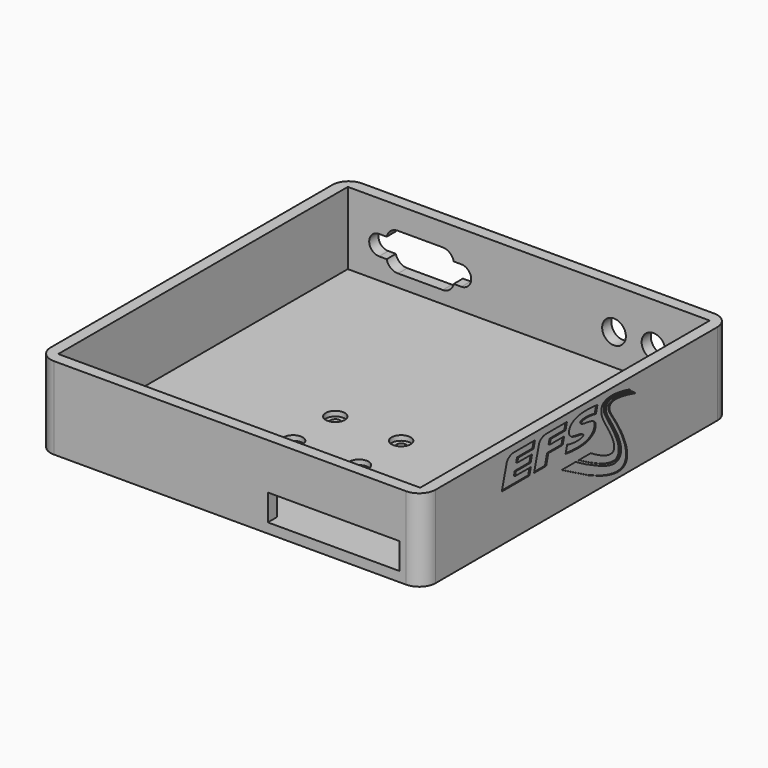
from build123d import *

# Parameters (mm, degrees)
F0_W      = 117
F0_H      = 117
F0_W_2    = 110
F0_H_2    = 110
F1_DEPTH  = 25
F2_DEPTH  = 3
F3_R      = 5
F4_R      = 5
F5_R      = 5
F7_R      = 3.6
F8_DEPTH  = 8.5856
F9_W      = 40
F9_H      = 8
F10_DEPTH = 25
F11_R     = 1.5
F12_DEPTH = 3
F13_R     = 2.9
F14_DEPTH = 1.5
F17_DEPTH = 2
F18_SCALE = 0.2


# Not quite as in the source:
# - two fillets or chamfers of one size are made in one step
# - a feature names something its author has since deleted; it is built from what else it names


with BuildPart() as f1:
    # F0 (on Top) → F1 (new body)
    with BuildSketch(Plane.XY):
        with Locations((0, 23.8324391609)):
            Rectangle(F0_W, F0_H)
        with Locations((0, 23.8324391609)):
            Rectangle(F0_W_2, F0_H_2, mode=Mode.SUBTRACT)
    extrude(amount=F1_DEPTH)

    # F0 (on Top) → F2 (join)
    with BuildSketch(Plane.XY):
        with Locations((0, 23.8324391609)):
            Rectangle(F0_W_2, F0_H_2)
    extrude(amount=F2_DEPTH)

    # F3
    f3_edges = [f1.edges().sort_by_distance(p)[0] for p in [
        (58.5, -34.667561, 12.5),
    ]]
    fillet(f3_edges, radius=F3_R)

    # F4
    f4_edges = [f1.edges().sort_by_distance(p)[0] for p in [
        (-58.5, -34.667561, 12.5),
    ]]
    fillet(f4_edges, radius=F4_R)

    # F5
    f5_edges = [f1.edges().sort_by_distance(p)[0] for p in [
        (58.5, 82.332439, 12.5),
        (-58.5, 82.332439, 12.5),
    ]]
    fillet(f5_edges, radius=F5_R)

    # F7 (on face) → F8 (cut)
    with BuildSketch(Plane(origin=(0, 82.3324391609, 0), x_dir=(-1, 0, 0), z_dir=(0, 1, 0))):
        with BuildLine():
            Line((39.85, 18.2), (26.15, 18.2))
            ThreePointArc((26.15, 18.2), (24.0075714714, 17.4400757565), (22.8228390481, 15.5))
            Line((22.8228390481, 15.5), (20.5, 15.5))
            ThreePointArc((20.5, 15.5), (17.5, 12.5), (20.5, 9.5))
            Line((20.5, 9.5), (22.8228390481, 9.5))
            ThreePointArc((22.8228390481, 9.5), (24.0075714714, 7.5599242435), (26.15, 6.8))
            Line((26.15, 6.8), (39.7201597989, 6.8))
            ThreePointArc((39.7201597989, 6.8), (41.9426174229, 7.5177900105), (43.1776817724, 9.5))
            Line((43.1776817724, 9.5), (45.5, 9.5))
            ThreePointArc((45.5, 9.5), (48.5, 12.5), (45.5, 15.5))
            ThreePointArc((45.5, 15.5), (44.2542750291, 15.2291334333), (43.2335002222, 14.465446198))
            ThreePointArc((43.2335002222, 14.465446198), (43.2449696229, 14.984881744), (43.1771609519, 15.5))
            ThreePointArc((43.1771609519, 15.5), (41.9924285286, 17.4400757565), (39.85, 18.2))
        make_face()
        with BuildLine():
            Line((45.5, 15.5), (43.1771609519, 15.5))
            ThreePointArc((43.1771609519, 15.5), (43.2449696229, 14.984881744), (43.2335002222, 14.465446198))
            ThreePointArc((43.2335002222, 14.465446198), (44.2542750291, 15.2291334333), (45.5, 15.5))
        make_face()
        with Locations((-37.9, 12.5)):
            Circle(F7_R)
        with Locations((-25.9, 12.5)):
            Circle(F7_R)
    extrude(amount=-F8_DEPTH, mode=Mode.SUBTRACT)

    # F9 (on face) → F10 (cut)
    with BuildSketch(Plane.XZ.offset(34.6675608391)):
        with Locations((31.5, 7)):
            Rectangle(F9_W, F9_H)
    extrude(amount=-F10_DEPTH, mode=Mode.SUBTRACT)

    # F11 (on face) → F12 (cut, through all)
    with BuildSketch(Plane(origin=(0, 0, 0), x_dir=(1, 0, 0), z_dir=(0, 0, -1))):
        with Locations((-10, -1.8324391609)):
            Circle(F11_R)
        with Locations((10, -1.8324391609)):
            Circle(F11_R)
        with Locations((10, -17.8324391609)):
            Circle(F11_R)
        with Locations((-10, -17.8324391609)):
            Circle(F11_R)
    extrude(amount=-F12_DEPTH, mode=Mode.SUBTRACT)

    # F13 (on face) → F14 (cut)
    with BuildSketch(Plane.XY.offset(3)):
        with Locations((-10, 17.8324391609)):
            Circle(F13_R)
        with Locations((10, 17.8324391609)):
            Circle(F13_R)
        with Locations((10, 1.8324391609)):
            Circle(F13_R)
        with Locations((-10, 1.8324391609)):
            Circle(F13_R)
    extrude(amount=-F14_DEPTH, mode=Mode.SUBTRACT)


with BuildPart() as f17:
    # F16 (on face) → F17 (new body)
    with BuildSketch(Plane.YZ.offset(58.5)):
        Polygon((-66.8057338, 42.572559), (-64.087883, 52.9304758), (-103.1221458, 52.9304758), (-105.1262312, 52.8319492), (-106.9472588, 52.599463), (-108.5937376, 52.2488668), (-110.0742782, 51.7959594), (-111.397415, 51.2566158), (-112.0026462, 50.9594866), (-112.5717078, 50.6466856), (-113.1057174, 50.3201686), (-113.605691, 49.9819676), (-114.5079498, 49.2783368), (-115.2869932, 48.5516174), (-115.9514064, 47.817659), (-116.5097492, 47.0922858), (-116.9705306, 46.3913728), (-117.3423612, 45.7307188), (-117.6337754, 45.1261988), (-117.8533076, 44.5936116), (-118.0095176, 44.1488576), (-127, 9.8964496), (-74.7851946, 9.8964496), (-72.0665818, 20.254341), (-101.9276346, 20.254341), (-100.3902996, 26.1122922), (-72.406383, 26.1122922), (-69.6877702, 36.469447), (-97.6724742, 36.469447), (-96.0704454, 42.572559), align=None)
    extrude(amount=F17_DEPTH)


with BuildPart() as f17b:
    # F16 (on face) → F17, piece 2 (new body)
    with BuildSketch(Plane.YZ.offset(58.5)):
        Polygon((-43.0960671327, 52.859241217), (-44.9142245327, 52.685556017), (-46.5680947327, 52.396834217), (-48.0652977327, 52.007071217), (-49.4133773327, 51.530287817), (-50.6199281327, 50.980530217), (-51.6925193327, 50.371819217), (-52.6387455327, 49.718175617), (-53.4661759327, 49.033620217), (-54.1824051327, 48.332199217), (-54.7950023327, 47.627908017), (-55.3115113327, 46.934818217), (-55.7395775327, 46.266925217), (-56.0867193327, 45.638275217), (-56.3605567327, 45.062863617), (-56.5686335327, 44.554736617), (-56.7185697327, 44.127940417), (-65.7222855327, 9.825215017), (-42.8577135327, 9.825215017), (-38.8280543327, 25.176848017), (-11.5263309327, 25.176848017), (-8.8073371327, 35.534764817), (-36.1094669327, 35.534764817), (-34.2811749327, 42.501324417), (-6.1265957327, 42.501324417), (-3.4072463327, 52.859241217), align=None)
    extrude(amount=F17_DEPTH)


with BuildPart() as f17c:
    # F16 (on face) → F17, piece 3 (new body)
    with BuildSketch(Plane.YZ.offset(58.5)):
        Polygon((24.8065699738, 38.5670330833), (24.6279825738, 38.6749830833), (24.4689531738, 38.7889782833), (24.3967917738, 38.8482110833), (24.3295071738, 38.9089678833), (24.2670993738, 38.9712486833), (24.2096191738, 39.0350026833), (24.1569903738, 39.1002806833), (24.1092891738, 39.1670826833), (24.0664647738, 39.2353832833), (24.0285425738, 39.3051824833), (23.9955225738, 39.3764802833), (23.9673793738, 39.4493020833), (23.9441383738, 39.5236224833), (23.9257995738, 39.5994668833), (23.9123629738, 39.6768098833), (23.9038285738, 39.7556768833), (23.9001709738, 39.8360424833), (23.9014155738, 39.9179320833), (23.9075877738, 40.0013202833), (23.9186367738, 40.0862070833), (23.9345879738, 40.1726432833), (23.9554413738, 40.2605526833), (23.9932111738, 40.3896608833), (24.0379913738, 40.5149336833), (24.0897565738, 40.6363456833), (24.1485321738, 40.7538968833), (24.2143181738, 40.8676126833), (24.2870891738, 40.9774930833), (24.3668705738, 41.0835126833), (24.4536623738, 41.1856714833), (24.5474391738, 41.2839948833), (24.6482009738, 41.3784574833), (24.7559731738, 41.4690846833), (24.8707303738, 41.5558510833), (24.9924725738, 41.6387820833), (25.1212251738, 41.7178522833), (25.3996853738, 41.8644610833), (26.0093107738, 42.1243538833), (26.6684153738, 42.3495502833), (27.3769483738, 42.5401010833), (28.1349351738, 42.6961332833), (29.7398849738, 42.9194754833), (31.4237271738, 43.0355280833), (34.5112241738, 43.0971992833), (39.2403993738, 42.9508698833), (43.6999789738, 42.5110942833), (47.8392899738, 41.8248878833), (51.6060337738, 40.9386056833), (54.5020909738, 51.9749310833), (45.0174515738, 53.0544056833), (35.1828509738, 53.4551160833), (29.9537529738, 53.3236710833), (24.5078659738, 52.9303012833), (21.7730733738, 52.6089150833), (19.1244375738, 52.1679710833), (16.5618823738, 51.6074438833), (14.0852553738, 50.9272064833), (11.7318437738, 50.1083104833), (9.5396967738, 49.1313248833), (8.5041641738, 48.5835738833), (7.5090175738, 47.9963258833), (6.5542823738, 47.3696316833), (5.6400093738, 46.7034658833), (4.7826323738, 45.9910974833), (4.0008711738, 45.2257954833), (3.2946749738, 44.4075598833), (2.6640437738, 43.5363398833), (2.1089013738, 42.6121608833), (1.6292731738, 41.6349720833), (1.2251083738, 40.6047988833), (0.8963815738, 39.5215904833), (0.7153049738, 38.7507004833), (0.5850029738, 38.0106968833), (0.5054247738, 37.3015542833), (0.4766211738, 36.6233234833), (0.4985413738, 35.9759536833), (0.5712107738, 35.3594702833), (0.6265827738, 35.0627982833), (0.6946293738, 34.7738478833), (0.7753505738, 34.4926190833), (0.8687463738, 34.2191118833), (1.0837827738, 33.6900298833), (1.3298325738, 33.1822584833), (1.6068449738, 32.6957722833), (1.9147691738, 32.2304950833), (2.2535543738, 31.7863760833), (2.6231497738, 31.3634152833), (3.0235045738, 30.9615364833), (3.4545425738, 30.5806888833), (3.9142571738, 30.2205422833), (4.3989653738, 29.8796234833), (4.9086671738, 29.5579832833), (5.4433625738, 29.2555962833), (6.5877849738, 28.7086580833), (7.8322833738, 28.2389612833), (10.4708099738, 27.4446524833), (13.2100729738, 26.7894086833), (18.7191551738, 25.8336574833), (23.4991303738, 25.0322620833), (24.4765477738, 24.8047542833), (25.3467517738, 24.5542340833), (26.1094629738, 24.2808030833), (26.7644527738, 23.9845374833), (26.9089787738, 23.9054418833), (27.0418461738, 23.8225108833), (27.1630549738, 23.7357444833), (27.2726051738, 23.6451426833), (27.3704967738, 23.5507054833), (27.4567297738, 23.4524582833), (27.4954647738, 23.4018868833), (27.5313041738, 23.3503502833), (27.5641971738, 23.2978484833), (27.5941945738, 23.2444068833), (27.6212455738, 23.1900000833), (27.6454009738, 23.1346280833), (27.6666353738, 23.0783162833), (27.6849487738, 23.0210392833), (27.7003411738, 22.9627970833), (27.7128125738, 22.9035896833), (27.7223375738, 22.8434170833), (27.7289669738, 22.7823046833), (27.7326753738, 22.7202270833), (27.7334627738, 22.6571842833), (27.7262491738, 22.5282284833), (27.7073261738, 22.3954372833), (27.6767191738, 22.2588106833), (27.6473821738, 22.1593188833), (27.6118475738, 22.0618082833), (27.5701407738, 21.9662788833), (27.5222617738, 21.8726798833), (27.4682105738, 21.7810620833), (27.4079871738, 21.6914000833), (27.3415915738, 21.6036684833), (27.2690745738, 21.5178926833), (27.1903853738, 21.4340726833), (27.1055493738, 21.3522084833), (26.9174877738, 21.1942712833), (26.7048897738, 21.0440556833), (26.4678315738, 20.9015870833), (25.9364635738, 20.6358268833), (25.3422051738, 20.3931552833), (24.6847515738, 20.1735976833), (23.9637725738, 19.9772302833), (22.3662903738, 19.6608478833), (20.5849121738, 19.4531774833), (16.6619583738, 19.2991772833), (11.5255703738, 19.4761644833), (6.3540033738, 20.0078626833), (1.4031115738, 20.8934082833), (-0.8934040262, 21.4696580833), (-3.0704634262, 22.1350618833), (-5.9986770262, 10.9753940833), (5.7966511738, 9.4342998833), (18.0384859738, 8.9412858833), (23.0822401738, 9.1030838833), (28.3184247738, 9.5886810833), (30.9387903738, 9.9717638833), (33.4677667738, 10.4742520833), (35.9055317738, 11.0965012833), (38.2521869738, 11.8388416833), (40.4787255738, 12.7152686833), (42.5582743738, 13.7420128833), (44.4909349738, 14.9193536833), (45.4021599738, 15.5645898833), (46.2766819738, 16.2476212833), (47.0970003738, 16.9722070833), (47.8456399738, 17.7440622833), (48.5226515738, 18.5631868833), (49.1280351738, 19.4296316833), (49.6618161738, 20.3433458833), (50.1240199738, 21.3043294833), (50.5146719738, 22.3126078833), (50.8337721738, 23.3681810833), (51.0618895738, 24.3752402833), (51.2047137738, 25.3313724833), (51.2622447738, 26.2364760833), (51.2590189738, 26.6699016833), (51.2344571738, 27.0905510833), (51.1885847738, 27.4984242833), (51.1213509738, 27.8935212833), (51.0327557738, 28.2758166833), (50.9228499738, 28.6453358833), (50.7915827738, 29.0020534833), (50.6389541738, 29.3459694833), (50.4649641738, 29.6770584833), (50.2696127738, 29.9953458833), (49.8343583738, 30.6023296833), (49.3526727738, 31.1745916833), (48.8245305738, 31.7121826833), (48.2499825738, 32.2151026833), (47.6289779738, 32.6833516833), (46.9615421738, 33.1169296833), (46.2477005738, 33.5158366833), (45.4874023738, 33.8800980833), (43.8729021738, 34.5273916833), (42.1652601738, 35.0821784833), (40.3644255738, 35.5444330833), (38.4704999738, 35.9142062833), (31.2194095738, 37.0549964833), (28.1587095738, 37.5870248833), (25.7163725738, 38.1954056833), (25.4596039738, 38.2793018833), (25.2223679738, 38.3691924833), (25.0046899738, 38.4651028833), align=None)
    extrude(amount=F17_DEPTH)


with BuildPart() as f17d:
    # F16 (on face) → F17, piece 4 (new body)
    with BuildSketch(Plane.YZ.offset(58.5)):
        Polygon((96.6154782211, -29.5210946531), (96.7791304211, -28.6497984531), (96.9000852211, -27.7165262531), (96.9769964211, -26.7194746531), (97.0116166211, -25.5120856531), (96.9890106211, -24.3224512531), (96.7878172211, -21.9947190531), (96.4049630211, -19.7328744531), (95.8719694211, -17.5335392531), (94.4816242211, -13.3086810531), (92.8690290211, -9.2928394531), (89.1307332211, -1.1737548531), (85.0315288211, 6.5280331469), (76.2592832211, 21.7010279469), (74.1142278211, 25.3788717469), (71.6841336211, 29.8454617469), (70.5762618211, 32.1975017469), (69.6540132211, 34.5342509469), (69.2892438211, 35.6747871469), (69.0030112211, 36.7849195469), (68.8059834211, 37.8558597469), (68.7442868211, 38.3738419469), (68.7089046211, 38.8786923469), (68.6925470211, 39.9895359469), (68.7439058211, 41.0324091469), (68.8602378211, 42.0093185469), (69.0386728211, 42.9223469469), (69.2764676211, 43.7735263469), (69.5708028211, 44.5649395469), (69.9188844211, 45.2986439469), (70.3179438211, 45.9766461469), (70.7651616211, 46.6010543469), (71.2577438211, 47.1739005469), (71.7929218211, 47.6972167469), (72.3678508211, 48.1731111469), (72.9797876211, 48.6035903469), (73.6259128211, 48.9907371469), (74.3034324211, 49.3365835469), (75.0095270211, 49.6432123469), (75.7414534211, 49.9126555469), (76.4963922211, 50.1469705469), (78.0641056211, 50.5184455469), (79.6903406211, 50.7740965469), (81.3527198211, 50.9303319469), (84.6964774211, 51.0103927469), (87.9165370211, 50.8900729469), (94.2782464211, 50.2470719469), (101.2295406211, 49.1073231469), (114.4758946211, 46.0586627469), (119.0977040211, 44.7786297469), (115.1308590211, 47.9630023469), (111.8250998211, 48.9000083469), (103.3942048211, 50.9196893469), (92.0676336211, 52.8350271469), (86.0151946211, 53.3826257469), (83.0136004211, 53.4890009469), (80.0748712211, 53.4590289469), (77.2338558211, 53.2741423469), (74.5254030211, 52.9158245469), (71.9842854211, 52.3654827469), (70.7874120211, 52.0125497469), (69.6454280211, 51.6046257469), (68.5627022211, 51.1394501469), (67.5435780211, 50.6146861469), (66.5924496211, 50.0279969469), (65.7136350211, 49.3770965469), (65.3027138211, 49.0268305469), (64.9115030211, 48.6596481469), (64.5405614211, 48.2752445469), (64.1904224211, 47.8733403469), (63.8616194211, 47.4536307469), (63.5547112211, 47.0158363469), (63.2702312211, 46.5596777469), (63.0087382211, 46.0848501469), (62.7707656211, 45.5910741469), (62.5568722211, 45.0780195469), (62.3675914211, 44.5454577469), (62.2034566211, 43.9930839469), (62.0650266211, 43.4205679469), (61.9528602211, 42.8276811469), (61.8674654211, 42.2140679469), (61.8094264211, 41.5794997469), (61.7774732211, 40.2462029469), (61.8614202211, 38.8255301469), (62.0655854211, 37.3151191469), (62.3943376211, 35.7126585469), (62.8520202211, 34.0158115469), (63.4429766211, 32.2223175469), (65.0422114211, 28.3359397469), (67.2268146211, 24.0350339469), (70.0316858211, 19.3010327469), (77.0650474211, 7.5259229469), (81.9961018211, -2.0739308531), (83.7355446211, -6.1135722531), (85.0241120211, -9.6759984531), (85.8867214211, -12.7833328531), (86.1660706211, -14.1732970531), (86.3482648211, -15.4578004531), (86.4364028211, -16.6396370531), (86.4336342211, -17.7215754531), (86.3991156211, -18.2259432531), (86.3430324211, -18.7063842531), (86.2657656211, -19.1632286531), (86.1677216211, -19.5968574531), (86.0492814211, -20.0075754531), (85.9108260211, -20.3957382531), (85.7527618211, -20.7617014531), (85.5754698211, -21.1058206531), (85.3793310211, -21.4284260531), (85.1647264211, -21.7298732531), (84.9320624211, -22.0104924531), (84.6817200211, -22.2706646531), (84.4141056211, -22.5106946531), (84.1296002211, -22.7309634531), (83.8285848211, -22.9318012531), (83.5114404211, -23.1135636531), (83.1785734211, -23.2765808531), (82.8303648211, -23.4212084531), (82.4671956211, -23.5478020531), (82.0894722211, -23.6567172531), (81.6975756211, -23.7482588531), (81.2918868211, -23.8228332531), (80.4407328211, -23.9223250531), (79.5391344211, -23.9579612531), (78.5901396211, -23.9325358531), (77.5969488211, -23.8488174531), (76.5625846211, -23.7096000531), (74.3829852211, -23.2756410531), (72.0761826211, -22.6528838531), (69.6671450211, -21.8635026531), (64.6418566211, -19.8736666531), (59.5063068211, -17.4836028531), (49.7012972211, -12.2128742531), (41.8456868211, -7.4713800531), (18.7105794211, -7.4971102531), (24.8572270211, -10.9724398531), (42.6591980211, -20.7908860531), (59.4668098211, -28.8970166531), (69.1033412211, -32.8239328531), (74.2499146211, -34.5645440531), (76.8742680211, -35.2843546531), (79.5208464211, -35.8677418531), (82.6988690211, -36.3923026531), (84.2530696211, -36.5688326531), (85.7693226211, -36.6691372531), (87.2365790211, -36.6788908531), (88.6437390211, -36.5838186531), (89.3213348211, -36.4925056531), (89.9797536211, -36.3695950531), (90.6176238211, -36.2133342531), (91.2335484211, -36.0219198531), (91.8261812211, -35.7935738531), (92.3940998211, -35.5264674531), (92.9359326211, -35.2188734531), (93.4503080211, -34.8689884531), (93.9358290211, -34.4749836531), (94.3911240211, -34.0351064531), (94.8147960211, -33.5475534531), (95.2054734211, -33.0105466531), (95.5617592211, -32.4223080531), (95.8822818211, -31.7810088531), (96.1656696211, -31.0849218531), (96.4105256211, -30.3321928531), align=None)
    extrude(amount=F17_DEPTH)


with BuildPart() as f17e:
    # F16 (on face) → F17, piece 5 (new body)
    with BuildSketch(Plane.YZ.offset(58.5)):
        Polygon((96.7758360174, 44.9829962893), (101.8384116174, 44.2651668893), (111.9346322174, 42.2222702893), (127.0185746174, 38.2900200893), (121.8416990174, 42.4422850893), (111.0816240174, 45.3691524893), (100.4274162174, 47.7687412893), (95.2388820174, 48.6361766893), (90.1954580174, 49.2102166893), (85.3367174174, 49.4370386893), (82.9889446174, 49.4034090893), (80.7021826174, 49.2627946893), (79.7957836174, 49.1581720893), (78.8800374174, 48.9997522893), (77.9649262174, 48.7831410893), (77.0603306174, 48.5038934893), (76.1761820174, 48.1576406893), (75.3224118174, 47.7399884893), (74.9100174174, 47.5029810893), (74.5089514174, 47.2464918893), (74.1204330174, 46.9699366893), (73.7456814174, 46.6727820893), (73.3860174174, 46.3544692893), (73.0426094174, 46.0144648893), (72.7167020174, 45.6521846893), (72.4095652174, 45.2670952893), (72.1224436174, 44.8586632893), (71.8565310174, 44.4263298893), (71.6131228174, 43.9695108893), (71.3934382174, 43.4876982893), (71.1986964174, 42.9803332893), (71.0301674174, 42.4468570893), (70.8890704174, 41.8867108893), (70.7766500174, 41.2993612893), (70.6941762174, 40.6842748893), (70.6428428174, 40.0408420893), (70.6239198174, 39.3685802893), (70.6386518174, 38.6668798893), (70.6823652174, 38.1326670893), (70.7640770174, 37.5718604893), (71.0276274174, 36.3886268893), (71.4015662174, 35.1536534893), (71.8581820174, 33.9033384893), (72.9084720174, 31.5025304893), (73.9565776174, 29.4777694893), (85.7422284174, 9.6670140893), (91.3165378174, -0.4996407107), (93.8601700174, -5.8669909107), (96.1790630174, -11.5069847107), (97.8296058174, -16.3940971107), (98.5806076174, -19.3206597107), (99.1340990174, -22.4335313107), (99.3021200174, -24.0280417107), (99.3791074174, -25.6309595107), (99.3512690174, -27.2295847107), (99.2046602174, -28.8111665107), (98.9254380174, -30.3630049107), (98.7317630174, -31.1238111107), (98.4997340174, -31.8723999107), (98.2276238174, -32.6071711107), (97.9136798174, -33.3265753107), (97.5561748174, -34.0290123107), (97.1533816174, -34.7128565107), (97.0245528174, -34.9010959107), (96.8656504174, -35.1084615107), (96.4720774174, -35.5669315107), (95.4826712174, -36.5626115107), (94.4157950174, -37.4801357107), (93.9253972174, -37.8408665107), (93.7035536174, -37.9847321107), (93.5021062174, -38.0996671107), (93.0516118174, -38.3208757107), (92.5875538174, -38.5222215107), (91.6203218174, -38.8669757107), (90.6037376174, -39.1372317107), (89.5411540174, -39.3363169107), (88.4358984174, -39.4675333107), (87.2913236174, -39.5341829107), (86.1107316174, -39.5395931107), (84.8975006174, -39.4870405107), (82.3864312174, -39.2213311107), (79.7848362174, -38.7635215107), (74.4167748174, -37.3775959107), (69.0070574174, -35.5409473107), (63.7693488174, -33.4653609107), (54.6645918174, -29.4444139107), (33.3166284174, -18.9967081107), (13.0282768174, -7.4924639107), (-13.7202853826, -7.4807545107), (37.7219028174, -35.4461545107), (57.6973264174, -44.3227179107), (66.2834662174, -47.5620307107), (73.9852288174, -50.0538723107), (80.8401300174, -51.8371555107), (86.8856856174, -52.9507677107), (89.6166682174, -53.2685979107), (92.1593860174, -53.4335963107), (94.5185380174, -53.4506397107), (96.6987724174, -53.3245541107), (98.7048136174, -53.0602163107), (100.5413352174, -52.6625031107), (101.3974930174, -52.4151579107), (102.2130362174, -52.1362659107), (102.9885490174, -51.8264621107), (103.7245902174, -51.4863561107), (104.4217948174, -51.1165575107), (105.0807216174, -50.7176505107), (105.7019548174, -50.2902701107), (106.2860786174, -49.8350259107), (106.8336772174, -49.3525021107), (107.3453602174, -48.8433083107), (107.8216864174, -48.3080541107), (108.2632400174, -47.7473745107), (108.6706560174, -47.1618537107), (109.0444678174, -46.5520759107), (109.3852850174, -45.9187015107), (109.6936664174, -45.2623147107), (109.9702470174, -44.5834997107), (110.2155602174, -43.8828915107), (110.6148228174, -42.4187085107), (110.8961532174, -40.8746425107), (111.0642504174, -39.2554941107), (111.1237626174, -37.5661909107), (111.0794142174, -35.8115589107), (110.9358788174, -33.9964495107), (110.6978554174, -32.1257649107), (109.9571152174, -28.2370249107), (108.8946332174, -24.1842517107), (107.5479760174, -20.0063073107), (104.1521484174, -11.4305561107), (100.0697080174, -2.8208705107), (91.0453166174, 13.2555768893), (82.8755590174, 25.7337840893), (80.9526774174, 28.6378930893), (79.4657614174, 31.2646594893), (78.8788182174, 32.4776364893), (78.3925098174, 33.6256148893), (78.0040168174, 34.7100170893), (77.7106214174, 35.7322908893), (77.5094534174, 36.6938840893), (77.3977950174, 37.5962444893), (77.3746556174, 38.0256314893), (77.3728268174, 38.4407690893), (77.3919784174, 38.8418096893), (77.4317802174, 39.2289564893), (77.4918512174, 39.6023618893), (77.5718358174, 39.9622036893), (77.6714292174, 40.3086850893), (77.7902504174, 40.6419838893), (77.9279692174, 40.9622778893), (78.0842300174, 41.2697194893), (78.2586518174, 41.5645118893), (78.4509298174, 41.8468582893), (78.6607338174, 42.1168856893), (78.8876574174, 42.3748226893), (79.1313704174, 42.6208470893), (79.3915680174, 42.8550858893), (79.6678438174, 43.0777676893), (79.9598676174, 43.2890702893), (80.2673092174, 43.4891714893), (80.5898130174, 43.6782236893), (81.2785848174, 44.0239684893), (82.0233890174, 44.3277778893), (82.8214824174, 44.5910742893), (83.6700456174, 44.8152800893), (84.5662846174, 45.0018938893), (85.5074562174, 45.1522872893), (87.5133196174, 45.3502802893), (89.6653854174, 45.4208414893), (91.9413778174, 45.3754516893), align=None)
    extrude(amount=F17_DEPTH)


with BuildPart() as f17_1:
    # F18: moved
    add(f17.part.scale(F18_SCALE).moved(Location((48.4, -89.117932, 41.00529264))))


with BuildPart() as f17b_1:
    # F18: moved
    add(f17b.part.scale(F18_SCALE).moved(Location((48.4, -89.117932, 41.00529264))))


with BuildPart() as f17c_1:
    # F18: moved
    add(f17c.part.scale(F18_SCALE).moved(Location((48.4, -89.117932, 41.00529264))))


with BuildPart() as f17d_1:
    # F18: moved
    add(f17d.part.scale(F18_SCALE).moved(Location((48.4, -89.117932, 41.00529264))))


with BuildPart() as f17e_1:
    # F18: moved
    add(f17e.part.scale(F18_SCALE).moved(Location((48.4, -89.117932, 41.00529264))))


with BuildPart() as f17_2:
    # F19: moved
    add(f17_1.part.moved(Location((-1.94668, 110, -28.7))))


with BuildPart() as f17b_2:
    # F19: moved
    add(f17b_1.part.moved(Location((-1.94668, 110, -28.7))))


with BuildPart() as f17c_2:
    # F19: moved
    add(f17c_1.part.moved(Location((-1.94668, 110, -28.7))))


with BuildPart() as f17d_2:
    # F19: moved
    add(f17d_1.part.moved(Location((-1.94668, 110, -28.7))))


with BuildPart() as f17e_2:
    # F19: moved
    add(f17e_1.part.moved(Location((-1.94668, 110, -28.7))))


with BuildPart() as f1_1:
    add(f1.part)

    # F20: cut F17, F17c, F17d, F17e, F17b
    add(f17_2.part, mode=Mode.SUBTRACT)
    add(f17c_2.part, mode=Mode.SUBTRACT)
    add(f17d_2.part, mode=Mode.SUBTRACT)
    add(f17e_2.part, mode=Mode.SUBTRACT)
    add(f17b_2.part, mode=Mode.SUBTRACT)


solid = f1_1.part
